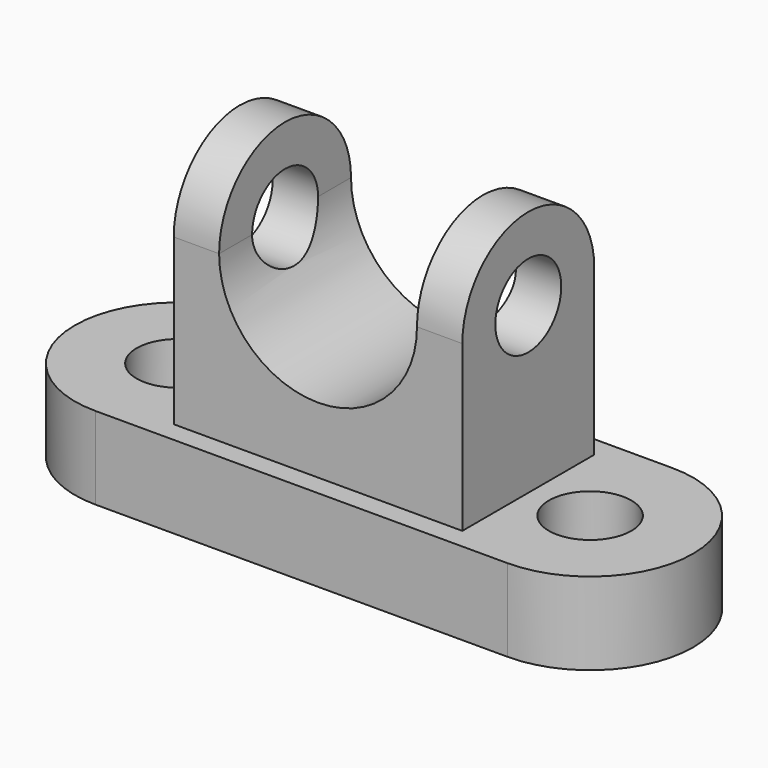
from build123d import *

# Parameters (mm, degrees)
F0_R     = 12.7
F1_DEPTH = 25.4
F2_W     = 88.9
F2_H     = 50.8
F3_DEPTH = 50.8
F5_DEPTH = 88.9
F7_DEPTH = 75.946
F8_R     = 12.7
F9_DEPTH = 112.776


# Not quite as in the source:
# - a feature names something its author has since deleted; it is built from what else it names


with BuildPart() as f1:
    # F0 (on Top) → F1 (new body)
    with BuildSketch(Plane.XY):
        with BuildLine():
            Line((-63.5, -31.75), (63.5, -31.75))
            ThreePointArc((63.5, -31.75), (95.25, 0), (63.5, 31.75))
            Line((63.5, 31.75), (-63.5, 31.75))
            ThreePointArc((-63.5, 31.75), (-95.25, 0), (-63.5, -31.75))
        make_face()
        with Locations((-63.5, 0)):
            Circle(F0_R, mode=Mode.SUBTRACT)
        with Locations((63.5, 0)):
            Circle(F0_R, mode=Mode.SUBTRACT)
    extrude(amount=F1_DEPTH)

    # F2 (on face) → F3 (join)
    with BuildSketch(Plane.XY.offset(25.4)):
        Rectangle(F2_W, F2_H)
    extrude(amount=F3_DEPTH)

    # F4 (on face) → F5 (join)
    with BuildSketch(Plane(origin=(-44.45, 0, 0), x_dir=(0, -1, 0), z_dir=(-1, 0, 0))):
        with BuildLine():
            Line((-25.4, 76.2), (25.4, 76.2))
            ThreePointArc((25.4, 76.2), (0, 101.6), (-25.4, 76.2))
        make_face()
    extrude(amount=-F5_DEPTH)

    # F6 (on face) → F7 (cut)
    with BuildSketch(Plane.XZ.offset(25.4)):
        with BuildLine():
            Line((-30.48, 76.2), (30.48, 76.2))
            ThreePointArc((30.48, 76.2), (0, 106.68), (-30.48, 76.2))
        make_face()
        with BuildLine():
            ThreePointArc((-30.48, 76.2), (0, 45.72), (30.48, 76.2))
            Line((30.48, 76.2), (-30.48, 76.2))
        make_face()
        with BuildLine():
            Line((30.48, 76.2), (30.48, 114.3))
            Line((30.48, 114.3), (-30.48, 114.3))
            Line((-30.48, 114.3), (-30.48, 76.2))
            ThreePointArc((-30.48, 76.2), (0, 106.68), (30.48, 76.2))
        make_face()
    extrude(amount=-F7_DEPTH, mode=Mode.SUBTRACT)

    # F8 (on face) → F9 (cut)
    with BuildSketch(Plane(origin=(-44.45, 0, 0), x_dir=(0, -1, 0), z_dir=(-1, 0, 0))):
        with Locations((0, 76.2)):
            Circle(F8_R)
    extrude(amount=-F9_DEPTH, mode=Mode.SUBTRACT)


solid = f1.part
